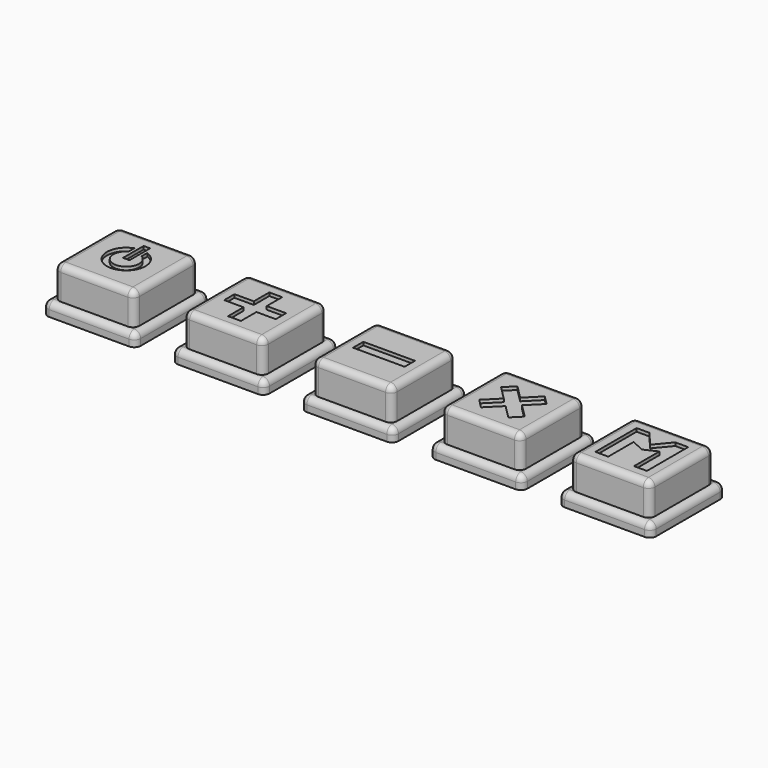
from build123d import *

# Parameters (mm, degrees)
F1_DEPTH  = 2.5
F2_R      = 1.7
F3_DEPTH  = 1
F4_DEPTH  = 0.5
F5_R      = 0.49999
F10_W     = 0.5
F10_H     = 2
F15_DEPTH = 0.25
F16_DEPTH = 0.25
F12_W     = 4
F12_H     = 1
F17_DEPTH = 0.25
F18_DEPTH = 0.25
F19_DEPTH = 0.25


# Not quite as in the source:
# - a fillet or chamfer is up to 0.001 mm smaller than in the source, because OpenCascade refuses the exact size


with BuildPart() as f1:
    # F0 (on Top) → F1 (new body)
    with BuildSketch(Plane.XY):
        with BuildLine():
            ThreePointArc((3.1, 2.6), (2.9535533906, 2.9535533906), (2.6, 3.1))
            Line((2.6, 3.1), (-2.6, 3.1))
            ThreePointArc((-2.6, 3.1), (-2.9535533906, 2.9535533906), (-3.1, 2.6))
            Line((-3.1, 2.6), (-3.1, -2.6))
            ThreePointArc((-3.1, -2.6), (-2.9535533906, -2.9535533906), (-2.6, -3.1))
            Line((-2.6, -3.1), (2.6, -3.1))
            ThreePointArc((2.6, -3.1), (2.9535533906, -2.9535533906), (3.1, -2.6))
            Line((3.1, -2.6), (3.1, 2.6))
        make_face()
    extrude(amount=F1_DEPTH)

    # F2 (on face) → F3 (join)
    with BuildSketch(Plane(origin=(0, 0, 0), x_dir=(1, 0, 0), z_dir=(0, 0, -1))):
        with BuildLine():
            ThreePointArc((3.6, 3.1), (3.4535533906, 3.4535533906), (3.1, 3.6))
            Line((3.1, 3.6), (-3.1, 3.6))
            ThreePointArc((-3.1, 3.6), (-3.4535533906, 3.4535533906), (-3.6, 3.1))
            Line((-3.6, 3.1), (-3.6, -3.1))
            ThreePointArc((-3.6, -3.1), (-3.4535533906, -3.4535533906), (-3.1, -3.6))
            Line((-3.1, -3.6), (3.1, -3.6))
            ThreePointArc((3.1, -3.6), (3.4535533906, -3.4535533906), (3.6, -3.1))
            Line((3.6, -3.1), (3.6, 3.1))
        make_face()
        Circle(F2_R, mode=Mode.SUBTRACT)
    extrude(amount=F3_DEPTH)

    # F4 (add): a face of the model
    f4_faces = [f1.faces().sort_by_distance(p)[0] for p in [
        (0, 0, 0),
    ]]
    extrude(f4_faces, amount=F4_DEPTH)

    # F5 (radius 0.5 in the source; OpenCascade refuses exactly that, so slightly less here)
    f5_edges = [f1.edges().sort_by_distance(p)[0] for p in [
        (3.1, 0, 2.5),
        (2.953553, 2.953553, 2.5),
        (0, 3.1, 2.5),
        (-2.953553, 2.953553, 2.5),
        (-3.1, 0, 2.5),
        (-2.953553, -2.953553, 2.5),
        (0, -3.1, 2.5),
        (2.953553, -2.953553, 2.5),
        (-3.6, 0, 0),
    ]]
    fillet(f5_edges, radius=F5_R)


with BuildPart() as f6_1:
    # F6: copy of F1
    add(f1.part.moved(Location((10, 0, 0))))


with BuildPart() as f7_1:
    # F7: copy of F6_1
    add(f6_1.part.moved(Location((10, 0, 0))))


with BuildPart() as f8_1:
    # F8: copy of F7_1
    add(f7_1.part.moved(Location((10, 0, 0))))


with BuildPart() as f9_1:
    # F9: copy of F8_1
    add(f8_1.part.moved(Location((10, 0, 0))))

    # F14 (on face) → F19 (cut)
    with BuildSketch(Plane.XY.offset(2.5)):
        Polygon((39, 2), (38, 2), (38, -2), (39, -2), (39, 0.4663076582), (40, 0), (41, 0.4663076582), (41, -2), (42, -2), (42, 2), (41, 2), (40, 0.8), align=None)
    extrude(amount=-F19_DEPTH, mode=Mode.SUBTRACT)


with BuildPart() as f1_1:
    add(f1.part)

    # F10 (on face) → F15 (cut)
    with BuildSketch(Plane.XY.offset(2.5)):
        with BuildLine():
            ThreePointArc((0.5, 0.8660254038), (0, -1), (-0.5, 0.8660254038))
            Line((-0.5, 0.8660254038), (-0.5, 1.4142135624))
            ThreePointArc((-0.5, 1.4142135624), (0, -1.5), (0.5, 1.4142135624))
            Line((0.5, 1.4142135624), (0.5, 0.8660254038))
        make_face()
        with Locations((0, 1)):
            Rectangle(F10_W, F10_H)
    extrude(amount=-F15_DEPTH, mode=Mode.SUBTRACT)


with BuildPart() as f6_1_1:
    add(f6_1.part)

    # F11 (on face) → F16 (cut)
    with BuildSketch(Plane.XY.offset(2.5)):
        Polygon((10.5, 2), (10, 2), (9.5, 2), (9.5, 0.5), (8, 0.5), (8, 0), (8, -0.5), (9.5, -0.5), (9.5, -2), (10, -2), (10.5, -2), (10.5, -0.5), (12, -0.5), (12, 0), (12, 0.5), (10.5, 0.5), align=None)
    extrude(amount=-F16_DEPTH, mode=Mode.SUBTRACT)


with BuildPart() as f7_1_1:
    add(f7_1.part)

    # F12 (on face) → F17 (cut)
    with BuildSketch(Plane.XY.offset(2.5)):
        with Locations((20, 0)):
            Rectangle(F12_W, F12_H)
    extrude(amount=-F17_DEPTH, mode=Mode.SUBTRACT)


with BuildPart() as f8_1_1:
    add(f8_1.part)

    # F13 (on face) → F18 (cut)
    with BuildSketch(Plane.XY.offset(2.5)):
        Polygon((31.767766953, 1.0606601718), (31.0606601718, 1.767766953), (30, 0.7071067812), (28.9393398282, 1.767766953), (28.232233047, 1.0606601718), (29.2928932188, 0), (28.232233047, -1.0606601718), (28.9393398282, -1.767766953), (30, -0.7071067812), (31.0606601718, -1.767766953), (31.767766953, -1.0606601718), (30.7071067812, 0), align=None)
    extrude(amount=-F18_DEPTH, mode=Mode.SUBTRACT)


solid = Compound([f9_1.part, f1_1.part, f6_1_1.part, f7_1_1.part, f8_1_1.part])
